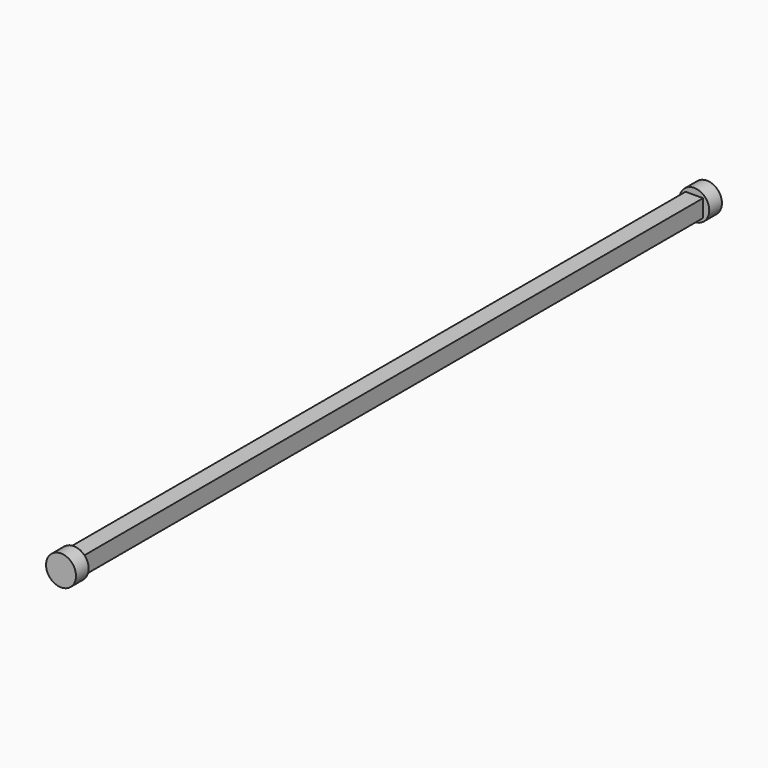
from build123d import *

# Parameters (mm, degrees)
F0_W          = 2.528925892
F0_H          = 2.5279636029
F1_DEPTH      = 56.0451
F1_DEPTH_BACK = 56.0451
F2_R          = 2.1639792623
F3_DEPTH      = 2.286


# Not quite as in the source:
# - a pattern or mirror of a feature is missing from the dataset's text; its kind, count and spacing are read off the source's solid


with BuildPart() as f1:
    # F0 (on Front) → F1 (new body, two sides)
    with BuildSketch(Plane.XZ) as f1_sk:
        Rectangle(F0_W, F0_H)
    extrude(amount=F1_DEPTH)
    extrude(f1_sk.sketch, amount=-F1_DEPTH_BACK)

    # F2 (on face) → F3 (join)
    with BuildSketch(Plane.XZ.offset(56.0451)):
        Circle(F2_R)
    f3 = extrude(amount=F3_DEPTH)

    # F3_copies: F3 across plane
    add(f3.mirror(Plane.ZX))


solid = f1.part
